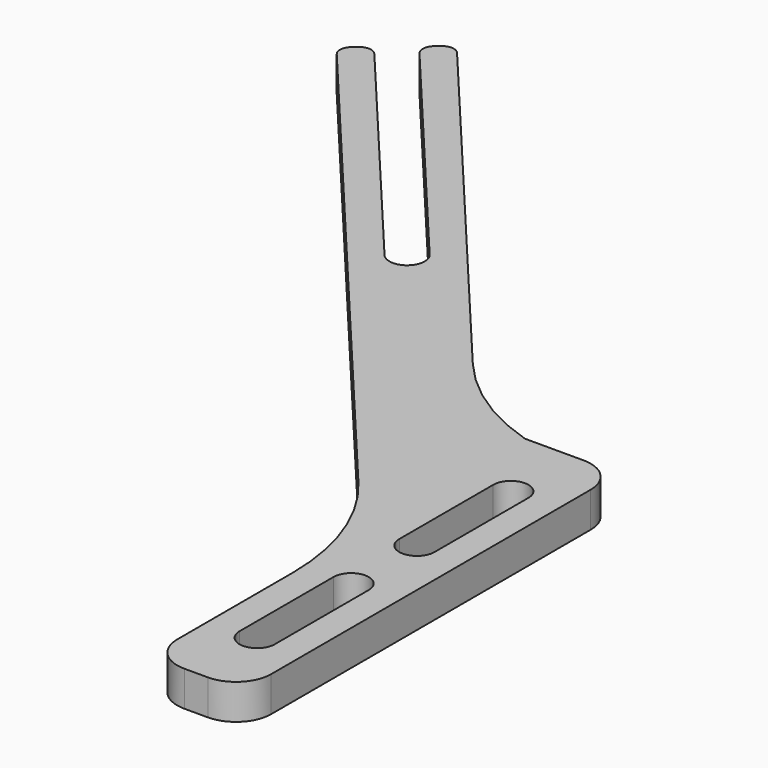
from build123d import *

# Parameters (mm, degrees)
F1_DEPTH    = 3
F2_R        = 1
F3_T1_DEPTH = 3
F4_R        = 3


# Not quite as in the source:
# - a fillet or chamfer that OpenCascade refuses, or shapes differently, is made with other operations: its cross-section is extruded or revolved along the edge and cut away or added


with BuildPart() as f1:
    # F0 (on Top) → F1 (new body)
    with BuildSketch(Plane.XY):
        with BuildLine():
            ThreePointArc((-29.4982599503, 56.7313189632), (-29.6831452005, 54.6180708839), (-31.7963932797, 54.8029561341))
            Line((-31.7963932797, 54.8029561341), (-51.0800215703, 77.7842894277))
            Line((-51.0800215703, 77.7842894277), (-52.9951326781, 76.1773204034))
            Line((-52.9951326781, 76.1773204034), (-8, 22.5542093851))
            Line((-8, 22.5542093851), (-8, 0))
            Line((-8, 0), (0, 0))
            Line((0, 0), (0, 40))
            Line((0, 40), (-8, 40))
            Line((-8, 40), (-8, 35))
            Line((-8, 35), (-46.8667771331, 81.3196212809))
            Line((-46.8667771331, 81.3196212809), (-48.7818882409, 79.7126522567))
            Line((-48.7818882409, 79.7126522567), (-29.4982599503, 56.7313189632))
        make_face()
        with BuildLine():
            Line((-2.5, 16.5), (-2.5, 6.5))
            ThreePointArc((-2.5, 6.5), (-4, 5), (-5.5, 6.5))
            Line((-5.5, 6.5), (-5.5, 16.5))
            ThreePointArc((-5.5, 16.5), (-4, 18), (-2.5, 16.5))
        make_face(mode=Mode.SUBTRACT)
        with BuildLine():
            Line((-2.5, 33.5), (-2.5, 23.5))
            ThreePointArc((-2.5, 23.5), (-4, 22), (-5.5, 23.5))
            Line((-5.5, 23.5), (-5.5, 33.5))
            ThreePointArc((-5.5, 33.5), (-4, 35), (-2.5, 33.5))
        make_face(mode=Mode.SUBTRACT)
    extrude(amount=F1_DEPTH)

    # F2
    f2_edges = [f1.edges().sort_by_distance(p)[0] for p in [
        (-52.995133, 76.17732, 1.5),
        (-51.080022, 77.784289, 1.5),
        (-48.781888, 79.712652, 1.5),
        (-46.866777, 81.319621, 1.5),
    ]]
    fillet(f2_edges, radius=F2_R)

    # F3: fillet of radius 20 on 2 edges, made by hand

    # F3_s2 → F3_t1 (join)
    with BuildSketch(Plane.XY):
        with BuildLine():
            ThreePointArc((-17.4512262706, 46.2635328624), (-13.1787684603, 42.4479872276), (-8, 40))
            Line((-8, 40), (-8, 35))
            Line((-8, 35), (-17.4512262706, 46.2635328624))
        make_face()
        with BuildLine():
            ThreePointArc((-8, 15.2748046998), (-9.2061475843, 22.1152075663), (-12.6791111376, 28.1305568935))
            Line((-12.6791111376, 28.1305568935), (-8, 22.5542093851))
            Line((-8, 22.5542093851), (-8, 15.2748046998))
        make_face()
    extrude(amount=F3_T1_DEPTH)

    # F4
    f4_edges = [f1.edges().sort_by_distance(p)[0] for p in [
        (0, 40, 1.5),
        (-8, 0, 1.5),
        (0, 0, 1.5),
    ]]
    fillet(f4_edges, radius=F4_R)


solid = f1.part
